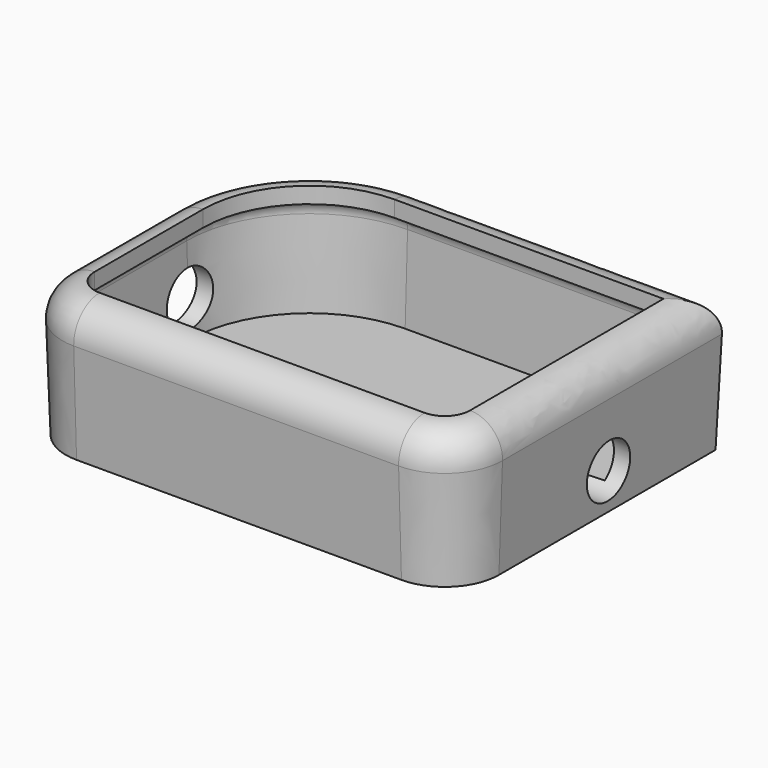
from build123d import *

# Parameters (mm, degrees)
F1_DEPTH = 25
F1_TAPER = -2
F2_R     = 6
F3_T     = 3
F5_D     = 10


# Not quite as in the source:
# - a shell that OpenCascade refuses in one call is made with other operations: the cavity is built on its own and cut out


with BuildPart() as f1:
    # F0 (on Top) → F1 (new body)
    with BuildSketch(Plane.XY):
        with BuildLine():
            Line((55, 25), (0, 25))
            ThreePointArc((0, 25), (-17.6776695297, 17.6776695297), (-25, 0))
            Line((-25, 0), (-25, -25))
            ThreePointArc((-25, -25), (-22.0710678119, -32.0710678119), (-15, -35))
            Line((-15, -35), (45, -35))
            ThreePointArc((45, -35), (52.0710678119, -32.0710678119), (55, -25))
            Line((55, -25), (55, 25))
        make_face()
    extrude(amount=F1_DEPTH, taper=F1_TAPER)

    # F2
    f2_edges = [f1.edges().sort_by_distance(p)[0] for p in [
        (15, -35.873019, 25),
    ]]
    fillet(f2_edges, radius=F2_R)

    # F3: shell of thickness 3, made by hand


with BuildPart() as f3_core1:
    # F3_t2: copy of F1
    add(f1.part)

    # the walls: a layer under each face that stays
    f3_faces = [f3_core1.faces().sort_by_distance(p)[0] for p in [
        (27.6640479465, 25.328095893, 9.3954370929),
        (-17.9096696286, 17.9096696286, 9.395488449),
        (27.794131329, 23.9760199568, 23.1679440438),
        (15, -5, 0),
        (55.3280962996, 0.1640481498, 9.3954487356),
        (-25.3280911583, -12.5, 9.3953015099),
        (-16.9638078754, 16.9431979233, 23.1679501064),
        (53.9760549891, 0.2869115749, 23.1679425379),
        (-22.3030632948, -32.3030632948, 9.3953015099),
        (15, -35.3280911583, 9.3953015099),
        (52.3030694739, -32.3030694739, 9.3955517523),
        (-23.9758761566, -12.5, 23.1679502228),
        (51.3377505062, -31.3560472609, 23.1679500628),
        (15, -33.9758761566, 23.1679502228),
        (-21.3469028974, -31.3469028974, 23.1679502228),
    ]]
    thicken(f3_faces, amount=-F3_T, mode=Mode.SUBTRACT)


with BuildPart() as f1_1:
    add(f1.part)

    # what is left inside the walls is the cavity
    f3_cavity = [f3_core1.part.solids().sort_by_distance(p)[0] for p in [
        (27.367645, -5, 3.03),
    ]]
    add(f3_cavity, mode=Mode.SUBTRACT)

    # F5 (through all)
    with Locations(Plane(origin=(54.9330113821, 0, -1.918303028), x_dir=(0, 1, 0), z_dir=(0.999390827, 0, -0.0348994967))):
        with Locations((0, 8.7753692642)):
            Hole(F5_D / 2)


solid = f1_1.part
